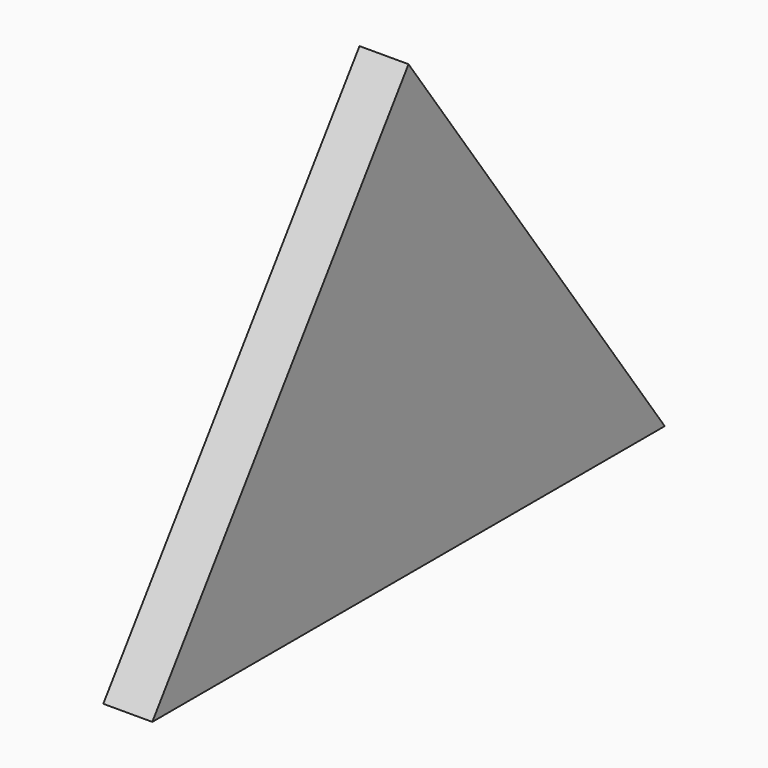
from build123d import *

# Parameters (mm, degrees)
F3_DEPTH = 5


# Not quite as in the source:
# - the program builds the solid bodies; features that only make, move or delete a surface that nothing else refers to are left out


with BuildPart() as f3:
    # F2 (on Right) → F3 (new body)
    with BuildSketch(Plane.YZ):
        Polygon((-32.6684378088, 4.2884717695), (0, 4.2884717695), (0, 50.0715896487), align=None)
        Polygon((0, 50.0715896487), (0, 4.2884717695), (32.6684378088, 4.2884717695), align=None)
    extrude(amount=F3_DEPTH)


solid = f3.part
